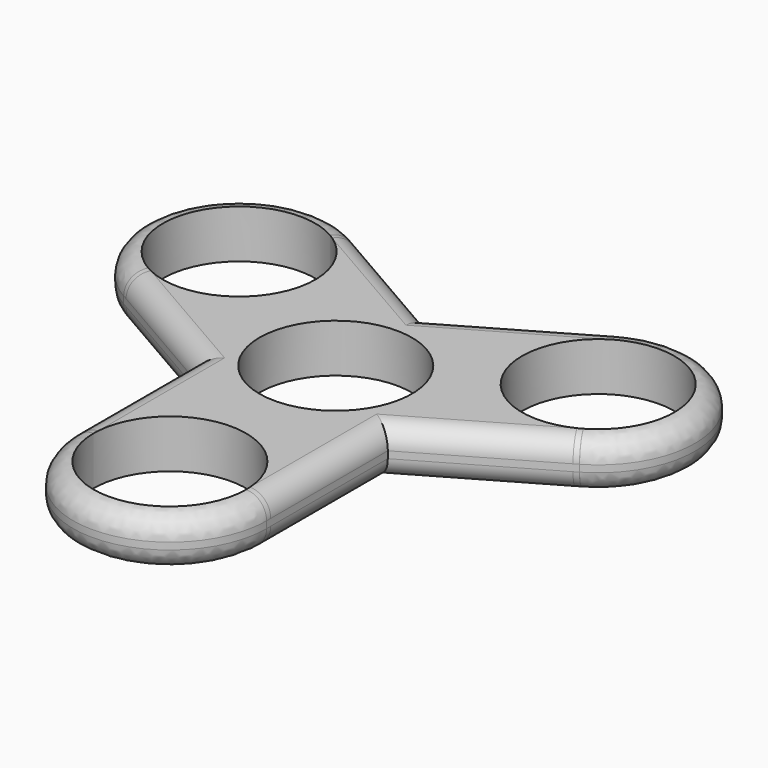
from build123d import *

# Parameters (mm, degrees)
F1_DEPTH        = 177.8
F1_COPIES_COUNT = 3
F3_R            = 76.2


# Not quite as in the source:
# - a feature of the source that left no trace in its solid (it failed there, or was rolled back) is left out
# - a pattern or mirror of a feature is missing from the dataset's text; its kind, count and spacing are read off the source's solid


with BuildPart() as f1:
    # F0 (on Top) → F1 (new body)
    with BuildSketch(Plane.XY):
        with BuildLine():
            Line((711.2, 0), (635.635, 0))
            ThreePointArc((635.635, 0), (355.6, -280.035), (75.565, 0))
            Line((75.565, 0), (0, 0))
            ThreePointArc((0, 0), (355.6, -355.6), (711.2, 0))
        make_face()
        with BuildLine():
            ThreePointArc((75.565, 0), (355.6, 280.035), (635.635, 0))
            Line((635.635, 0), (711.2, 0))
            ThreePointArc((711.2, 0), (355.6, 355.6), (0, 0))
            Line((0, 0), (75.565, 0))
        make_face()
        with BuildLine():
            ThreePointArc((0, 0), (355.6, 355.6), (711.2, 0))
            Line((711.2, 0), (711.2, 762))
            ThreePointArc((711.2, 762), (355.6, 406.4), (0, 762))
            Line((0, 762), (0, 0))
        make_face()
        with BuildLine():
            Line((635.635, 762), (711.2, 762))
            ThreePointArc((711.2, 762), (355.6, 1117.6), (0, 762))
            Line((0, 762), (75.565, 762))
            ThreePointArc((75.565, 762), (355.6, 1042.035), (635.635, 762))
        make_face()
        with BuildLine():
            ThreePointArc((0, 762), (355.6, 406.4), (711.2, 762))
            Line((711.2, 762), (635.635, 762))
            ThreePointArc((635.635, 762), (355.6, 481.965), (75.565, 762))
            Line((75.565, 762), (0, 762))
        make_face()
    extrude(amount=F1_DEPTH)

    # F1_copies: F1 ×3 about axis
    f1_copies_axis = Axis((355.6, 762, 0), (0, 0, 1))


with BuildPart() as f1_1:
    add(f1.part)
    for i in range(1, F1_COPIES_COUNT):
        add(f1.part.rotate(f1_copies_axis, i * 360 / F1_COPIES_COUNT))

    # F3
    f3_edges = [f1_1.edges().sort_by_distance(p)[0] for p in [
        (0, 278.347122, 177.8),
        (0, 278.347122, 0),
        (711.2, 278.347122, 177.8),
        (711.2, 278.347122, 0),
        (355.6, -355.6, 177.8),
        (355.6, -355.6, 0),
        (596.655679, 1311.785073, 177.8),
        (114.544321, 1311.785073, 177.8),
        (-241.055679, 695.867805, 177.8),
        (952.255679, 695.867805, 177.8),
        (952.255679, 695.867805, 0),
        (-241.055679, 695.867805, 0),
        (114.544321, 1311.785073, 0),
        (596.655679, 1311.785073, 0),
    ]]
    fillet(f3_edges, radius=F3_R)


solid = f1_1.part
